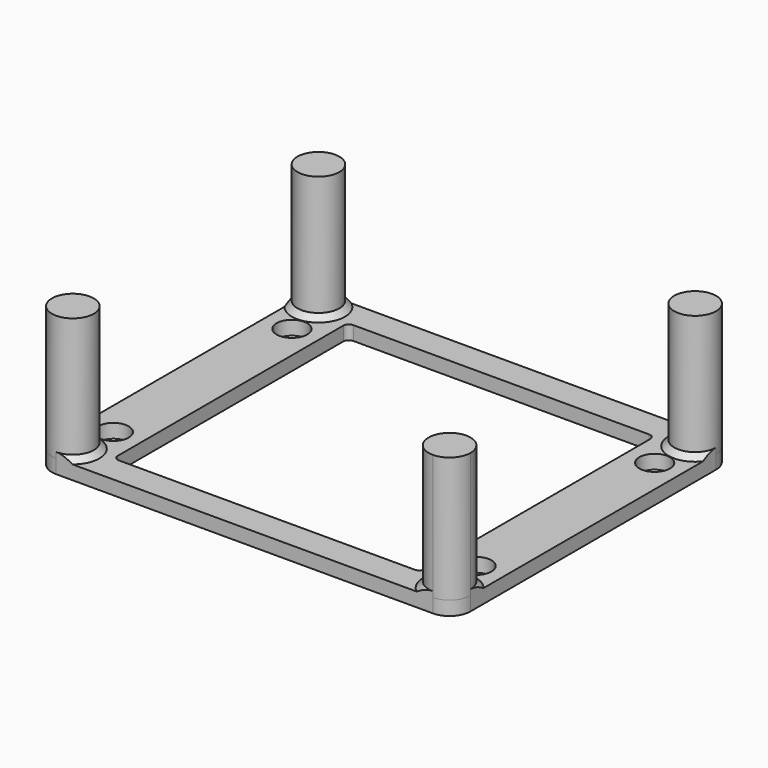
from build123d import *

# Parameters (mm, degrees)
F0_W         = 110
F0_H         = 105
F1_DEPTH     = 5
F2_DEPTH     = 45
F3_D         = 11
F4_R         = 7.4999
F5_R         = 2
F6_T4_ANGLE  = 270.0000001091
F6_T10_ANGLE = 270
F6_T16_ANGLE = 269.9999994391
F6_T22_ANGLE = 270


# Not quite as in the source:
# - a fillet or chamfer that OpenCascade refuses, or shapes differently, is made with other operations: its cross-section is extruded or revolved along the edge and cut away or added
# - a fillet or chamfer is up to 0.001 mm smaller than in the source, because OpenCascade refuses the exact size


with BuildPart() as f1:
    # F0 (on Top) → F1 (new body)
    with BuildSketch(Plane.XY):
        with BuildLine():
            Line((-73.2421757894, 65.9002404553), (-80.7421757894, 65.9002404553))
            Line((-80.7421757894, 65.9002404553), (-80.7421757894, 58.4002404553))
            ThreePointArc((-80.7421757894, 58.4002404553), (-78.5454766483, 63.7035413142), (-73.2421757894, 65.9002404553))
        make_face()
        with BuildLine():
            Line((61.7578242249, 65.9002404553), (-73.2421757894, 65.9002404553))
            ThreePointArc((-73.2421757894, 65.9002404553), (-67.9388749305, 63.7035413142), (-65.7421757894, 58.4002404553))
            ThreePointArc((-65.7421757894, 58.4002404553), (-73.2421757894, 50.9002404553), (-80.7421757894, 58.4002404553))
            Line((-80.7421757894, 58.4002404553), (-80.7421757894, -51.5997595447))
            ThreePointArc((-80.7421757894, -51.5997595447), (-73.2421757894, -44.0997595447), (-65.7421757894, -51.5997595447))
            ThreePointArc((-65.7421757894, -51.5997595447), (-67.9388749305, -56.9030604036), (-73.2421757894, -59.0997595447))
            Line((-73.2421757894, -59.0997595447), (61.757824248, -59.0997595447))
            ThreePointArc((61.757824248, -59.0997595447), (56.4545233385, -46.296458699), (69.2578242106, -51.5997595447))
            Line((69.2578242106, -51.5997595447), (69.2578242106, 58.4002404553))
            ThreePointArc((69.2578242106, 58.4002404553), (56.4545233466, 53.0969396015), (61.7578242249, 65.9002404553))
        make_face()
        with Locations((-5.7421757894, 3.4002404553)):
            Rectangle(F0_W, F0_H, mode=Mode.SUBTRACT)
        with BuildLine():
            Line((69.2578242106, 65.9002404553), (61.7578242249, 65.9002404553))
            ThreePointArc((61.7578242249, 65.9002404553), (67.0611250745, 63.7035413092), (69.2578242106, 58.4002404553))
            Line((69.2578242106, 58.4002404553), (69.2578242106, 65.9002404553))
        make_face()
        with BuildLine():
            ThreePointArc((61.757824248, -59.0997595447), (67.0611250827, -56.9030603903), (69.2578242106, -51.5997595447))
            ThreePointArc((69.2578242106, -51.5997595447), (56.4545233385, -46.296458699), (61.757824248, -59.0997595447))
        make_face()
        with BuildLine():
            ThreePointArc((-65.7421757894, -51.5997595447), (-73.2421757894, -44.0997595447), (-80.7421757894, -51.5997595447))
            ThreePointArc((-80.7421757894, -51.5997595447), (-78.5454766483, -56.9030604036), (-73.2421757894, -59.0997595447))
            ThreePointArc((-73.2421757894, -59.0997595447), (-67.9388749305, -56.9030604036), (-65.7421757894, -51.5997595447))
        make_face()
        with BuildLine():
            ThreePointArc((69.2578242106, 58.4002404553), (67.0611250745, 63.7035413092), (61.7578242249, 65.9002404553))
            ThreePointArc((61.7578242249, 65.9002404553), (56.4545233466, 53.0969396015), (69.2578242106, 58.4002404553))
        make_face()
        with BuildLine():
            ThreePointArc((-65.7421757894, 58.4002404553), (-67.9388749305, 63.7035413142), (-73.2421757894, 65.9002404553))
            ThreePointArc((-73.2421757894, 65.9002404553), (-78.5454766483, 63.7035413142), (-80.7421757894, 58.4002404553))
            ThreePointArc((-80.7421757894, 58.4002404553), (-73.2421757894, 50.9002404553), (-65.7421757894, 58.4002404553))
        make_face()
        with BuildLine():
            ThreePointArc((-73.2421757894, -59.0997595447), (-78.5454766483, -56.9030604036), (-80.7421757894, -51.5997595447))
            Line((-80.7421757894, -51.5997595447), (-80.7421757894, -59.0997595447))
            Line((-80.7421757894, -59.0997595447), (-73.2421757894, -59.0997595447))
        make_face()
        with BuildLine():
            Line((69.2578242106, -59.0997595447), (69.2578242106, -51.5997595447))
            ThreePointArc((69.2578242106, -51.5997595447), (67.0611250827, -56.9030603903), (61.757824248, -59.0997595447))
            Line((61.757824248, -59.0997595447), (69.2578242106, -59.0997595447))
        make_face()
    extrude(amount=-F1_DEPTH)

    # F0 (on Top) → F2 (join)
    with BuildSketch(Plane.XY):
        with BuildLine():
            ThreePointArc((61.757824248, -59.0997595447), (67.0611250827, -56.9030603903), (69.2578242106, -51.5997595447))
            ThreePointArc((69.2578242106, -51.5997595447), (56.4545233385, -46.296458699), (61.757824248, -59.0997595447))
        make_face()
        with BuildLine():
            ThreePointArc((69.2578242106, 58.4002404553), (67.0611250745, 63.7035413092), (61.7578242249, 65.9002404553))
            ThreePointArc((61.7578242249, 65.9002404553), (56.4545233466, 53.0969396015), (69.2578242106, 58.4002404553))
        make_face()
        with BuildLine():
            ThreePointArc((-65.7421757894, -51.5997595447), (-73.2421757894, -44.0997595447), (-80.7421757894, -51.5997595447))
            ThreePointArc((-80.7421757894, -51.5997595447), (-78.5454766483, -56.9030604036), (-73.2421757894, -59.0997595447))
            ThreePointArc((-73.2421757894, -59.0997595447), (-67.9388749305, -56.9030604036), (-65.7421757894, -51.5997595447))
        make_face()
        with BuildLine():
            ThreePointArc((-65.7421757894, 58.4002404553), (-67.9388749305, 63.7035413142), (-73.2421757894, 65.9002404553))
            ThreePointArc((-73.2421757894, 65.9002404553), (-78.5454766483, 63.7035413142), (-80.7421757894, 58.4002404553))
            ThreePointArc((-80.7421757894, 58.4002404553), (-73.2421757894, 50.9002404553), (-65.7421757894, 58.4002404553))
        make_face()
    extrude(amount=F2_DEPTH)

    # F3 (through all)
    with Locations(Plane.XY):
        with Locations((-70.7421757894, 43.4002404553), (-70.7421757894, -36.5997595447), (59.2578242106, 43.4002404553), (59.2578242106, -36.5997595447)):
            Hole(F3_D / 2)

    # F4 (radius 7.5 in the source; OpenCascade refuses exactly that, so slightly less here)
    f4_edges = [f1.edges().sort_by_distance(p)[0] for p in [
        (69.257824, 65.90024, -2.5),
        (69.257824, -59.09976, -2.5),
        (-80.742176, -59.09976, -2.5),
        (-80.742176, 65.90024, -2.5),
    ]]
    fillet(f4_edges, radius=F4_R)

    # F5
    f5_edges = [f1.edges().sort_by_distance(p)[0] for p in [
        (-60.742176, 55.90024, -2.5),
        (49.257824, 55.90024, -2.5),
        (-60.742176, -49.09976, -2.5),
        (49.257824, -49.09976, -2.5),
    ]]
    fillet(f5_edges, radius=F5_R)

    # F6: chamfer of 2 on 4 edges, made by hand


with BuildPart() as f6_tool2:
    # F6_s3 → F6_t4 (revolve)
    with BuildSketch(Plane.YZ.offset(61.7578242106)):
        Polygon((67.9002404553, 0), (65.9002404553, 2), (65.9002404553, 0), align=None)
    revolve(axis=Axis((61.7578242106, 58.4002404553, 0), (0, 0, 1)), revolution_arc=F6_T4_ANGLE)

    split(bisect_by=Plane.XZ.offset(-65.9002404553), keep=Keep.TOP)

    split(bisect_by=Plane.YZ.offset(69.2578242106), keep=Keep.BOTTOM)


with BuildPart() as f1_1:
    add(f1.part)

    # F6_t1: union F6_tool2
    add(f6_tool2.part)


with BuildPart() as f6_tool8:
    # F6_s9 → F6_t10 (revolve)
    with BuildSketch(Plane.XZ.offset(-58.4002404553)):
        Polygon((-82.7421757894, 0), (-80.7421757894, 2), (-80.7421757894, 0), align=None)
    revolve(axis=Axis((-73.2421757894, 58.4002404553, 0), (0, 0, 1)), revolution_arc=F6_T10_ANGLE)

    split(bisect_by=Plane.YZ.offset(-80.7421757894), keep=Keep.TOP)

    split(bisect_by=Plane.XZ.offset(-65.9002404553), keep=Keep.TOP)


with BuildPart() as f1_2:
    add(f1_1.part)

    # F6_t7: union F6_tool8
    add(f6_tool8.part)


with BuildPart() as f6_tool14:
    # F6_s15 → F6_t16 (revolve)
    with BuildSketch(Plane.XZ.offset(51.5997595447)):
        Polygon((71.2578242106, 0), (69.2578242106, 2), (69.2578242106, 0), align=None)
    revolve(axis=Axis((61.7578242106, -51.5997595447, 0), (0, 0, 1)), revolution_arc=F6_T16_ANGLE)

    split(bisect_by=Plane.XZ.offset(59.0997595447), keep=Keep.BOTTOM)

    split(bisect_by=Plane.YZ.offset(69.2578242106), keep=Keep.BOTTOM)


with BuildPart() as f1_3:
    add(f1_2.part)

    # F6_t13: union F6_tool14
    add(f6_tool14.part)


with BuildPart() as f6_tool20:
    # F6_s21 → F6_t22 (revolve)
    with BuildSketch(Plane.YZ.offset(-73.2421757894)):
        Polygon((-61.0997595447, 0), (-59.0997595447, 2), (-59.0997595447, 0), align=None)
    revolve(axis=Axis((-73.2421757894, -51.5997595447, 0), (0, 0, 1)), revolution_arc=F6_T22_ANGLE)

    split(bisect_by=Plane.YZ.offset(-80.7421757894), keep=Keep.TOP)

    split(bisect_by=Plane.XZ.offset(59.0997595447), keep=Keep.BOTTOM)


with BuildPart() as f1_4:
    add(f1_3.part)

    # F6_t19: union F6_tool20
    add(f6_tool20.part)


solid = f1_4.part
